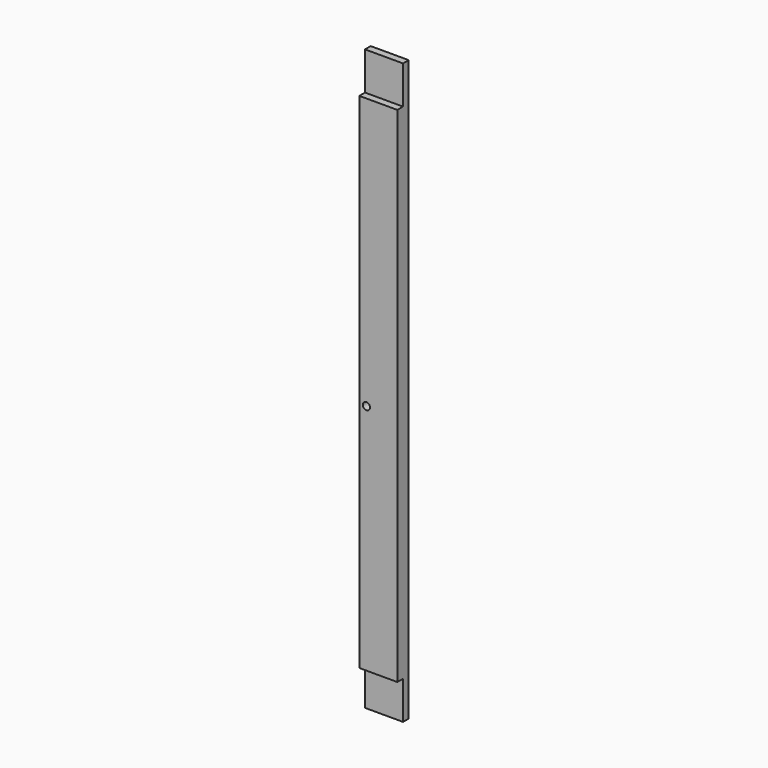
from build123d import *

# Parameters (mm, degrees)
F0_W     = 50.8
F0_H     = 19.05
F1_DEPTH = 774.7
F2_W     = 122.43557321
F2_H     = 50.8
F2_W_2   = 343.1604206562
F3_DEPTH = 25.4
F4_R     = 0.79375
F5_DEPTH = 25.4
F6_R     = 4.7625
F7_DEPTH = 25.4


# Not quite as in the source:
# - a feature names something its author has since deleted; it is built from what else it names


with BuildPart() as f1:
    # F0 (on Top) → F1 (new body)
    with BuildSketch(Plane.XY):
        Rectangle(F0_W, F0_H)
    extrude(amount=F1_DEPTH)

    # F2 (on Front) → F3 (cut)
    with BuildSketch(Plane.XZ):
        with Locations((22.4465244144, 25.4)):
            Rectangle(F2_W, F2_H)
        with Locations((-38.7818217278, 749.3)):
            Rectangle(F2_W_2, F2_H)
    extrude(amount=F3_DEPTH, mode=Mode.SUBTRACT)

    # F4 (on Front) → F5 (cut)
    with BuildSketch(Plane.XZ):
        with Locations((9.525, 101.6)):
            Circle(F4_R)
        with Locations((9.525, 155.575)):
            Circle(F4_R)
        with Locations((9.525, 619.125)):
            Circle(F4_R)
        with Locations((9.525, 673.1)):
            Circle(F4_R)
        with Locations((-9.525, 619.125)):
            Circle(F4_R)
        with Locations((-9.525, 673.1)):
            Circle(F4_R)
        with Locations((-9.525, 101.6)):
            Circle(F4_R)
        with Locations((-9.525, 155.575)):
            Circle(F4_R)
    extrude(amount=-F5_DEPTH, mode=Mode.SUBTRACT)

    # F6 (on Front) → F7 (cut)
    with BuildSketch(Plane.XZ):
        with Locations((-15.875, 361.95)):
            Circle(F6_R)
    extrude(amount=F7_DEPTH, mode=Mode.SUBTRACT)


solid = f1.part
